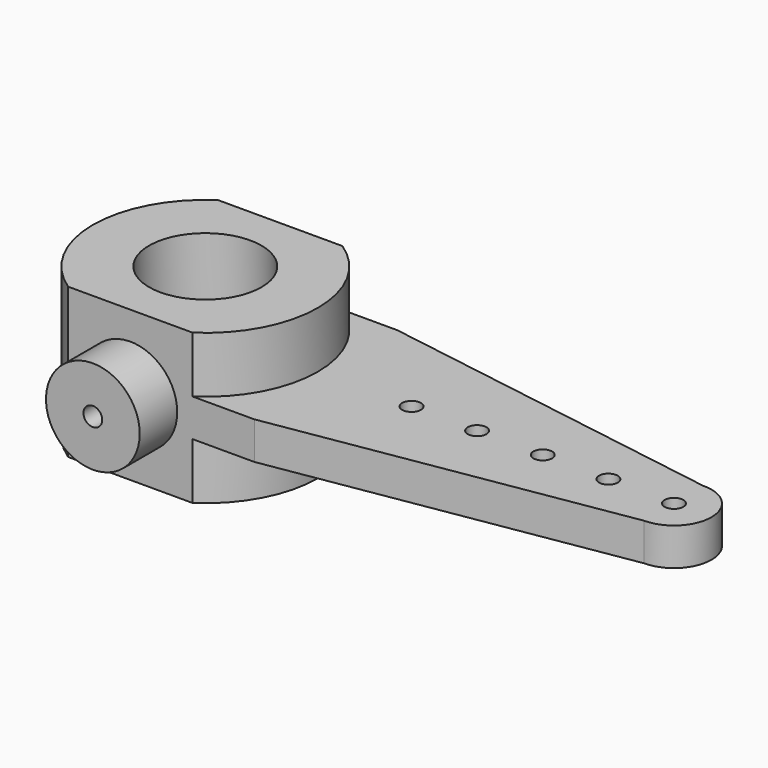
from build123d import *

# Parameters (mm, degrees)
F1_DEPTH = 4
F0_R     = 0.5
F2_DEPTH = 1
F3_R     = 2.5
F3_R_2   = 0.5
F4_DEPTH = 2.5


with BuildPart() as f1:
    # F0 (on Top) → F1 (new body, symmetric)
    with BuildSketch(Plane.XY):
        with BuildLine():
            Line((-3.3166247904, -5), (0, -5))
            Line((0, -5), (3.3166247904, -5))
            ThreePointArc((3.3166247904, -5), (6, 0), (3.3166247904, 5))
            Line((3.3166247904, 5), (-3.3166247904, 5))
            ThreePointArc((-3.3166247904, 5), (-6, 0), (-3.3166247904, -5))
        make_face()
        with BuildLine():
            ThreePointArc((0, -3), (-2.1213203436, 2.1213203436), (3, 0))
            ThreePointArc((3, 0), (2.1213203436, -2.1213203436), (0, -3))
        make_face(mode=Mode.SUBTRACT)
    extrude(amount=F1_DEPTH, both=True)

    # F0 (on Top) → F2 (join, symmetric)
    with BuildSketch(Plane.XY):
        with BuildLine():
            ThreePointArc((3.3166247904, 5), (6, 0), (3.3166247904, -5))
            Line((3.3166247904, -5), (6.6147298804, -5))
            Line((6.6147298804, -5), (25, -2))
            ThreePointArc((25, -2), (26.9998884615, 0.0211220617), (24.9577582326, 1.9995538585))
            Line((24.9577582326, 1.9995538585), (6.2387437176, 5))
            Line((6.2387437176, 5), (3.3166247904, 5))
        make_face()
        with Locations((11, 0)):
            Circle(F0_R, mode=Mode.SUBTRACT)
        with Locations((14.5, 0)):
            Circle(F0_R, mode=Mode.SUBTRACT)
        with Locations((18, 0)):
            Circle(F0_R, mode=Mode.SUBTRACT)
        with Locations((21.5, 0)):
            Circle(F0_R, mode=Mode.SUBTRACT)
        with Locations((25, 0)):
            Circle(F0_R, mode=Mode.SUBTRACT)
    extrude(amount=F2_DEPTH, both=True)

    # F3 (on face) → F4 (join)
    with BuildSketch(Plane.XZ.offset(5)):
        Circle(F3_R)
        Circle(F3_R_2, mode=Mode.SUBTRACT)
    extrude(amount=F4_DEPTH)


solid = f1.part
